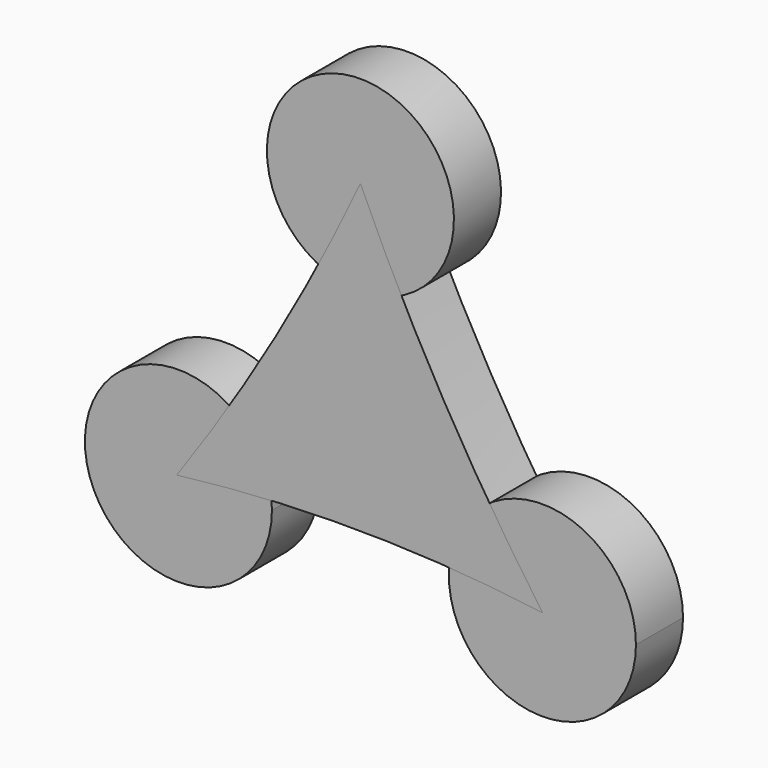
from build123d import *

# Parameters (mm, degrees)
F2_DEPTH = 7
F3_DEPTH = 7


# Not quite as in the source:
# - a feature of the source that left no trace in its solid (it failed there, or was rolled back) is left out


with BuildPart() as f2:
    # F0 (on Front) → F2 (new body)
    with BuildSketch(Plane.XZ):
        with BuildLine():
            ThreePointArc((9.6345326171, -5.5625), (10.7459248175, -2.8793618768), (11.125, 0))
            ThreePointArc((11.125, 0), (7.8665629407, 7.8665629407), (0, 11.125))
            Line((0, 11.125), (0, 0))
            Line((0, 0), (9.6345326171, -5.5625))
        make_face()
        with BuildLine():
            Line((0, 0), (0, 11.125))
            ThreePointArc((0, 11.125), (-9.6345326171, 5.5625), (-9.6345326171, -5.5625))
            Line((-9.6345326171, -5.5625), (0, 0))
        make_face()
        with BuildLine():
            ThreePointArc((-9.6345326171, -5.5625), (0, -11.125), (9.6345326171, -5.5625))
            Line((9.6345326171, -5.5625), (0, 0))
            Line((0, 0), (-9.6345326171, -5.5625))
        make_face()
    extrude(amount=F2_DEPTH)


with BuildPart() as f2b:
    # F0 (on Front) → F2, piece 2 (new body)
    with BuildSketch(Plane.XZ):
        with BuildLine():
            ThreePointArc((32.7756350946, -12.5), (24.5299969714, -1.7540751825), (12.0161024775, -6.9375))
            ThreePointArc((12.0161024775, -6.9375), (18.7712732178, -23.2459248175), (32.7756350946, -12.5))
        make_face()
    extrude(amount=F2_DEPTH)


with BuildPart() as f2c:
    # F0 (on Front) → F2, piece 3 (new body)
    with BuildSketch(Plane.XZ):
        with BuildLine():
            ThreePointArc((-10.5256350946, -12.5), (-10.9047102771, -9.6206381232), (-12.0161024775, -6.9375))
            ThreePointArc((-12.0161024775, -6.9375), (-32.3965599121, -15.3793618768), (-10.5256350946, -12.5))
        make_face()
    extrude(amount=F2_DEPTH)


with BuildPart() as f2d:
    # F0 (on Front) → F2, piece 4 (new body)
    with BuildSketch(Plane.XZ):
        with BuildLine():
            ThreePointArc((11.125, 25), (-7.8665629407, 32.8665629407), (0, 13.875))
            ThreePointArc((0, 13.875), (7.8665629407, 17.1334370593), (11.125, 25))
        make_face()
    extrude(amount=F2_DEPTH)


with BuildPart() as f3:
    # F1 (on Front) → F3 (new body)
    with BuildSketch(Plane.XZ):
        with BuildLine():
            ThreePointArc((0, 25.154441337), (-10.0854973849, 5.8528683876), (-21.8402211228, -12.480010428))
            ThreePointArc((-21.8402211228, -12.480010428), (-0.0723465521, -11.2352282244), (21.6776926373, -12.7602335754))
            ThreePointArc((21.6776926373, -12.7602335754), (9.9063592573, 5.6639549628), (0, 25.154441337))
        make_face()
    extrude(amount=F3_DEPTH)


solid = Compound([f2.part, f2b.part, f2c.part, f2d.part, f3.part])
